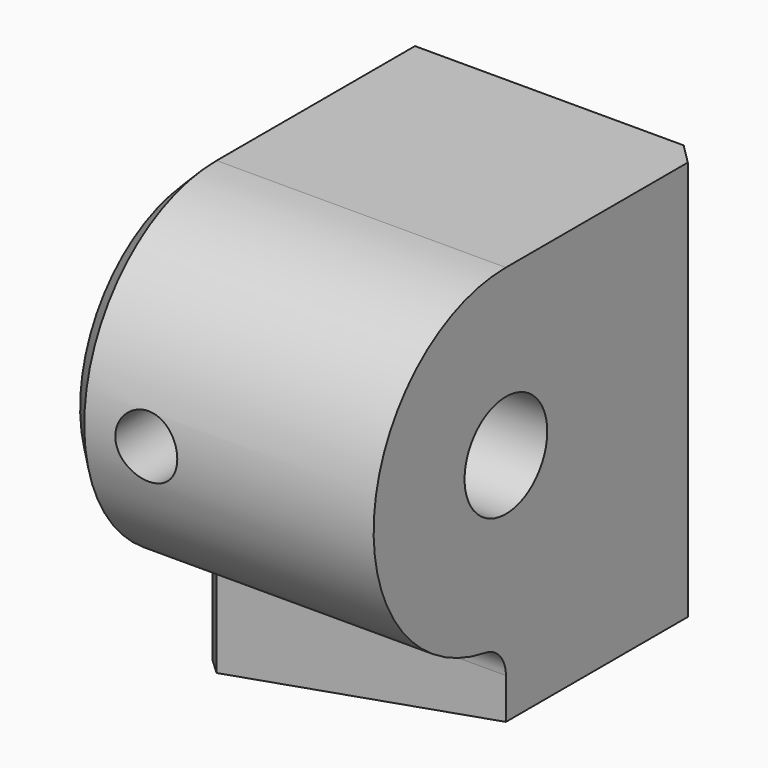
from build123d import *

# Parameters (mm, degrees)
F1_DEPTH       = 20
F3_D           = 5
F3_CBORE_D     = 9.75
F3_CBORE_DEPTH = 9.5
F5_D           = 4.5
F5_DEPTH       = 10
F5_TIP         = 1.3519363928
F6_R           = 1.5
F7_DEPTH       = 25
F9_DEPTH       = 15.001
F10_SIZE       = 1


with BuildPart() as f1:
    # F0 (on Front) → F1 (new body)
    with BuildSketch(Plane.XZ):
        Polygon((7.5, 0), (-7.5, 0), (-7.5, -22), (7.5, -19.3550952894), align=None)
    extrude(amount=-F1_DEPTH)

    # F3 (through all)
    with Locations(Plane(origin=(-7.5, 0, 0), x_dir=(0, -1, 0), z_dir=(-1, 0, 0))):
        with Locations((-8, -8)):
            CounterBoreHole(F3_D / 2, F3_CBORE_D / 2, F3_CBORE_DEPTH)

    # F5
    with Locations(Plane(origin=(3.5360689045, 0, -20.0540432912), x_dir=(0.984807753, 0, 0.1736481777), z_dir=(0.1736481777, 0, -0.984807753))):
        with Locations((-3.5906184671, -16)):
            Hole(F5_D / 2, depth=F5_DEPTH)
            with Locations((0, 0, -(F5_DEPTH + F5_TIP / 2))):  # 118° drill point
                Cone(0, F5_D / 2, F5_TIP, mode=Mode.SUBTRACT)

    # F6 (on face) → F7 (cut)
    with BuildSketch(Plane(origin=(0, 20, 0), x_dir=(-1, 0, 0), z_dir=(0, 1, 0))):
        with Locations((3.5, -8)):
            Circle(F6_R)
    extrude(amount=-F7_DEPTH, mode=Mode.SUBTRACT)

    # F8 (on face) → F9 (cut, through all)
    with BuildSketch(Plane(origin=(-7.5, 0, 0), x_dir=(0, -1, 0), z_dir=(-1, 0, 0))):
        with BuildLine():
            Line((0, 0), (-8, 0))
            ThreePointArc((-8, 0), (-2.3431457505, -2.3431457505), (0, -8))
            Line((0, -8), (0, 0))
        make_face()
        with BuildLine():
            Line((-8, -17.3808315196), (-8, -22))
            Line((-8, -22), (0, -22))
            Line((0, -22), (0, -8))
            ThreePointArc((0, -8), (-1.912912718, -13.1910854762), (-6.7368421053, -15.8996475955))
            ThreePointArc((-6.7368421053, -15.8996475955), (-7.6413288654, -16.4075029929), (-8, -17.3808315196))
        make_face()
    extrude(amount=-F9_DEPTH, mode=Mode.SUBTRACT)

    # F10
    f10_edges = [f1.edges().sort_by_distance(p)[0] for p in [
        (7.5, 20, -9.677548),
        (-7.5, 20, -11),
        (-7.5, 14, 0),
        (-7.5, 8, -19.690416),
        (-7.5, 12.875, -8),
        (-7.5, 7.641329, -16.407503),
        (-7.5, 0.025128, -7.366431),
    ]]
    chamfer(f10_edges, length=F10_SIZE)


solid = f1.part
